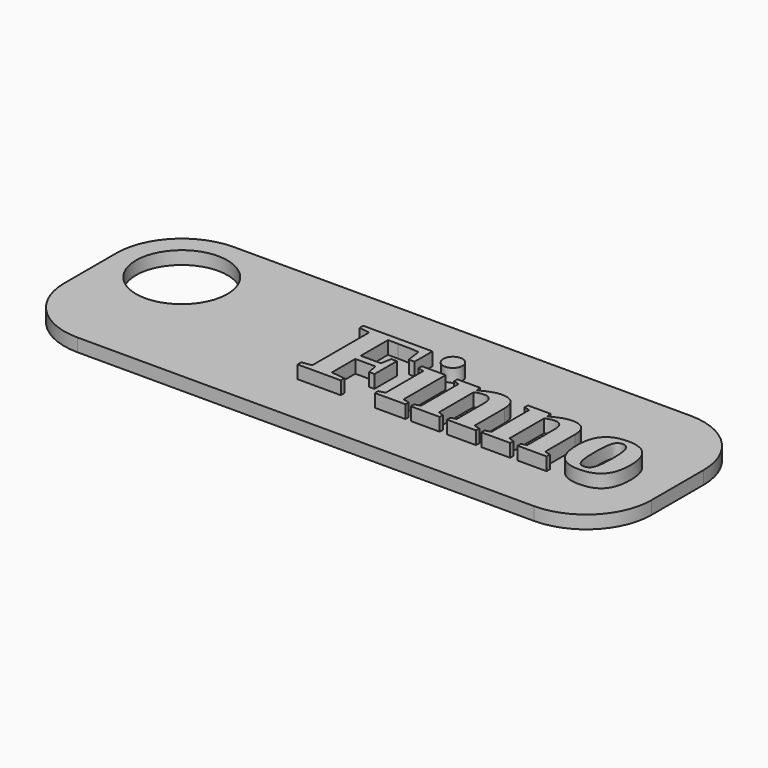
from build123d import *

# Parameters (mm, degrees)
F0_W         = 45
F0_H         = 15
F1_DEPTH     = 1
F2_R         = 5
F4_D         = 7
F4_DEPTH     = 15.5
F4_TIP       = 2.1030121666
F5_TEXT_SIZE = 9.7222222222
F6_DEPTH     = 1


# Not quite as in the source:
# - Text() gives the source's letters only with a copy of the font that has no kerning and outlines rounded to 1/6400 em; it was checked with that copy


with BuildPart() as f1:
    # F0 (on Top) → F1 (new body)
    with BuildSketch(Plane.XY):
        Rectangle(F0_W, F0_H)
    extrude(amount=F1_DEPTH)

    # F2
    f2_edges = [f1.edges().sort_by_distance(p)[0] for p in [
        (-22.5, -7.5, 0.5),
        (22.5, -7.5, 0.5),
        (22.5, 7.5, 0.5),
        (-22.5, 7.5, 0.5),
    ]]
    fillet(f2_edges, radius=F2_R)

    # F4
    with Locations(Plane.XY.offset(1)):
        with Locations((-17.5, 2.5)):
            Hole(F4_D / 2, depth=F4_DEPTH)
            with Locations((0, 0, -(F4_DEPTH + F4_TIP / 2))):  # 118° drill point
                Cone(0, F4_D / 2, F4_TIP, mode=Mode.SUBTRACT)

    # F5 (on face) → F6 (join)
    with BuildSketch(Plane.XY.offset(1)):
        with Locations((-4.0501302083, -3.5)):
            Text('Finno', F5_TEXT_SIZE, font='Tinos', font_style=FontStyle.BOLD, text_align=(TextAlign.LEFT, TextAlign.BOTTOM))
    extrude(amount=F6_DEPTH)


solid = f1.part
